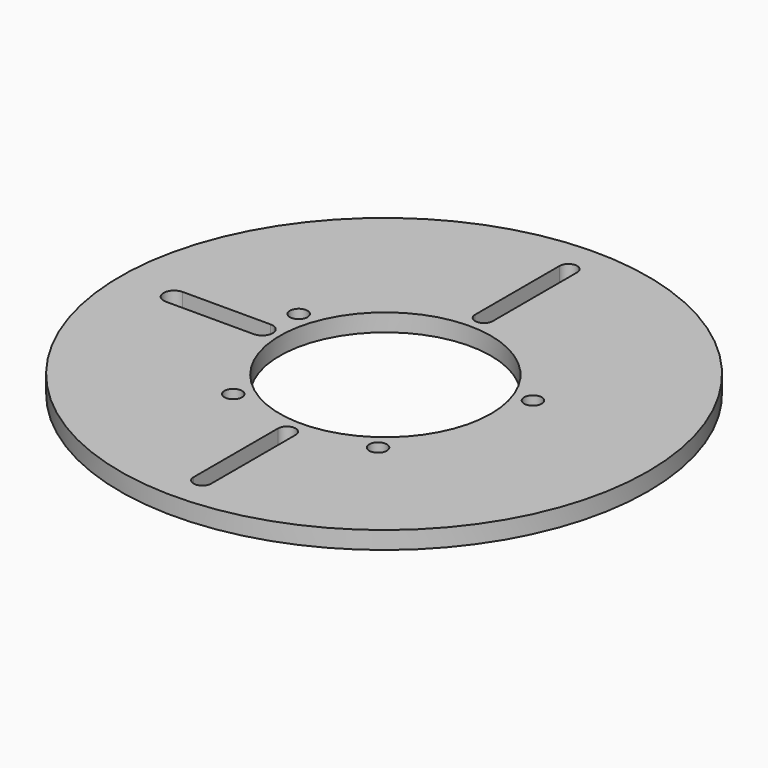
from build123d import *

# Parameters (mm, degrees)
F0_R     = 75
F0_R_2   = 30
F1_DEPTH = 5
F3_D     = 5
F5_DEPTH = 5
F7_DEPTH = 5


# Not quite as in the source:
# - a pattern or mirror of a feature is missing from the dataset's text; its kind, count and spacing are read off the source's solid


with BuildPart() as f1:
    # F0 (on Top) → F1 (new body)
    with BuildSketch(Plane.XY):
        with Locations((-0.4658745937, 0.1248266798)):
            Circle(F0_R)
        Circle(F0_R_2, mode=Mode.SUBTRACT)
    extrude(amount=F1_DEPTH)

    # F3 (through all)
    with Locations(Plane.XY.offset(5)):
        with Locations((0, 35), (33.2869780703, 10.8155948031), (20.5724838302, -28.3155948031), (-20.5724838302, -28.3155948031), (-33.2869780703, 10.8155948031)):
            Hole(F3_D / 2)

    # F4 (on face) → F5 (cut, through all)
    with BuildSketch(Plane.XY.offset(5)):
        with BuildLine():
            ThreePointArc((2.5, -35), (0, -32.5), (-2.5, -35))
            Line((-2.5, -35), (-2.5, -65))
            ThreePointArc((-2.5, -65), (0, -67.5), (2.5, -65))
            Line((2.5, -65), (2.5, -35))
        make_face()
    f5 = extrude(amount=-F5_DEPTH, mode=Mode.SUBTRACT)

    # F5_copies: F5 across plane
    add(f5.mirror(Plane.ZX), mode=Mode.SUBTRACT)

    # F6 (on face) → F7 (cut, through all)
    with BuildSketch(Plane.XY.offset(5)):
        with BuildLine():
            ThreePointArc((-60, 3), (-63, 0), (-60, -3))
            Line((-60, -3), (-35, -3))
            ThreePointArc((-35, -3), (-32, 0), (-35, 3))
            Line((-35, 3), (-60, 3))
        make_face()
    extrude(amount=-F7_DEPTH, mode=Mode.SUBTRACT)


solid = f1.part
